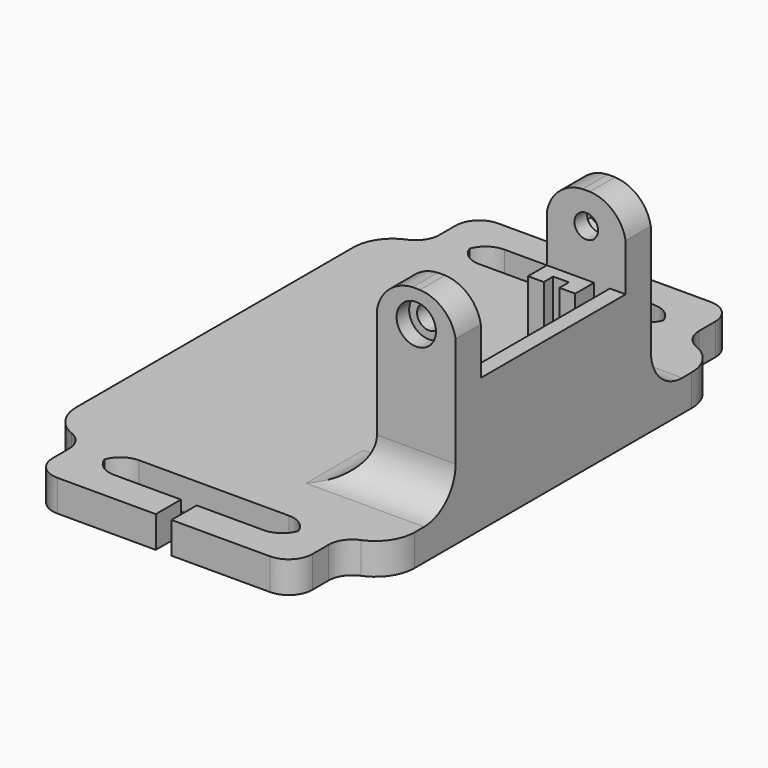
from build123d import *

# Parameters (mm, degrees)
F1_R          = 1.5
F2_DEPTH      = 4
F4_W          = 43
F4_H          = 54
F5_DEPTH      = 4
F6_R          = 5
F7_W          = 4
F7_H          = 4
F8_DEPTH      = 8
F8_DEPTH_BACK = 62
F9_W          = 4
F9_H          = 4
F10_DEPTH     = 25
F11_W         = 2
F11_H         = 4
F12_DEPTH     = 5
F11_H_2       = 15
F11_H_3       = 8
F11_H_4       = 1.5
F13_DEPTH     = 13
F14_DEPTH     = 7
F15_T1_DEPTH  = 3
F15_T3_DEPTH  = 3
F15_T5_DEPTH  = 2
F15_T7_DEPTH  = 4
F15_T12_DEPTH = 17
F15_T17_DEPTH = 17
F15_T22_DEPTH = 17
F15_T28_DEPTH = 9.5
F15_T33_DEPTH = 9.5
F15_T38_DEPTH = 17
F15_T45_DEPTH = 9.5
F15_T49_DEPTH = 10.5
F15_T56_DEPTH = 10.5
F15_T60_DEPTH = 9.5
F15_T63_DEPTH = 19
F16_R         = 2.5
F16_R_2       = 1.5
F17_DEPTH     = 2
F18_R         = 1.5
F19_DEPTH     = 2


# Not quite as in the source:
# - a fillet or chamfer that OpenCascade refuses, or shapes differently, is made with other operations: its cross-section is extruded or revolved along the edge and cut away or added


with BuildPart() as f2:
    # F1 (on offset) → F2 (new body)
    with BuildSketch(Plane.XZ.offset(11.5)):
        with BuildLine():
            Line((-10, 0), (0, 0))
            Line((0, 0), (0, 19))
            ThreePointArc((0, 19), (-1.5652731311, 21.7951628703), (-4.5336704997, 23))
            Line((-4.5336704997, 23), (-5, 23))
            Line((-5, 23), (-5.4663295003, 23))
            ThreePointArc((-5.4663295003, 23), (-8.4347268689, 21.7951628703), (-10, 19))
            Line((-10, 19), (-10, 0))
        make_face()
        with Locations((-5, 19)):
            Circle(F1_R, mode=Mode.SUBTRACT)
    extrude(amount=F2_DEPTH)


with BuildPart() as f3_1:
    # F3: instance of F2
    add(f2.part.mirror(Plane.XZ))


with BuildPart() as f2_1:
    add(f2.part)

    add(f3_1.part)  # F5 merges F3_1
    # F4 (on Top) → F5 (join)
    with BuildSketch(Plane.XY):
        with Locations((-21.5, 0)):
            Rectangle(F4_W, F4_H)
    extrude(amount=-F5_DEPTH)

    # F6
    f6_edges = [f2_1.edges().sort_by_distance(p)[0] for p in [
        (-5, -15.5, 0),
        (-5, 15.5, 0),
        (-10, 13.5, 0),
        (-10, -13.5, 0),
        (-43, 27, -2),
        (-43, -27, -2),
        (0, -27, -2),
        (0, 27, -2),
    ]]
    fillet(f6_edges, radius=F6_R)

    # F7 (on face) → F8 (join, two sides)
    with BuildSketch(Plane(origin=(0, 27, 0), x_dir=(-1, 0, 0), z_dir=(0, 1, 0))) as f8_sk:
        with Locations((36, -2)):
            Rectangle(F7_W, F7_H)
        with Locations((7, -2)):
            Rectangle(F7_W, F7_H)
    extrude(amount=F8_DEPTH)
    extrude(f8_sk.sketch, amount=-F8_DEPTH_BACK)

    # F9 (on face) → F10 (join)
    with BuildSketch(Plane.YZ.offset(-34)):
        with Locations((-33, -2)):
            Rectangle(F9_W, F9_H)
        with Locations((33, -2)):
            Rectangle(F9_W, F9_H)
    extrude(amount=F10_DEPTH)

    # F11 (on face) → F12 (cut)
    with BuildSketch(Plane.XY):
        with Locations((-21.5, -33)):
            Rectangle(F11_W, F11_H)
        with Locations((-21.5, 33)):
            Rectangle(F11_W, F11_H)
    extrude(amount=-F12_DEPTH, mode=Mode.SUBTRACT)

    # F11 (on face) → F13 (join)
    with BuildSketch(Plane.XY):
        with Locations((-1, 4)):
            Rectangle(F11_W, F11_H_2)
        with Locations((-1, -7.5)):
            Rectangle(F11_W, F11_H_3)
        Polygon((-6, -10), (-6, -11.5), (-4, -11.5), (-4, -8.5), (-6, -8.5), align=None)
        with Locations((-7, -10.75)):
            Rectangle(F11_W, F11_H_4)
        Polygon((-10, -8.5), (-10, -11.5), (-8, -11.5), (-8, -10), (-8, -8.5), align=None)
        Polygon((-8, 11.5), (-10, 11.5), (-10, 8.5), (-8, 8.5), (-8, 10), align=None)
        with Locations((-7, 10.75)):
            Rectangle(F11_W, F11_H_4)
        Polygon((-6, 8.5), (-4, 8.5), (-4, 11.5), (-6, 11.5), (-6, 10), align=None)
    extrude(amount=F13_DEPTH)

    # F11 (on face) → F14 (join)
    with BuildSketch(Plane.XY):
        Polygon((-4, -8.5), (-4, -11.5), (-2, -11.5), (-2, -3.5), (-2, 11.5), (-4, 11.5), (-4, 8.5), align=None)
    extrude(amount=F14_DEPTH)

    # F15: fillet of radius 3 on 22 edges, made by hand

    # F15_s2 → F15_t1 (join)
    with BuildSketch(Plane.XZ.offset(8.5)):
        with BuildLine():
            ThreePointArc((-13, 0), (-10.8786796564, 0.8786796564), (-10, 3))
            Line((-10, 3), (-10, 0))
            Line((-10, 0), (-13, 0))
        make_face()
    extrude(amount=F15_T1_DEPTH)

    # F15_s4 → F15_t3 (join)
    with BuildSketch(Plane.XZ.offset(-11.5)):
        with BuildLine():
            ThreePointArc((-13, 0), (-10.8786796564, 0.8786796564), (-10, 3))
            Line((-10, 3), (-10, 0))
            Line((-10, 0), (-13, 0))
        make_face()
    extrude(amount=F15_T3_DEPTH)

    # F15_s6 → F15_t5 (join)
    with BuildSketch(Plane.YZ.offset(-10)):
        with BuildLine():
            ThreePointArc((-5.5, 0), (-7.6213203436, 0.8786796564), (-8.5, 3))
            Line((-8.5, 3), (-8.5, 0))
            Line((-8.5, 0), (-5.5, 0))
        make_face()
        with BuildLine():
            ThreePointArc((5.5, 0), (7.6213203436, 0.8786796564), (8.5, 3))
            Line((8.5, 3), (8.5, 0))
            Line((8.5, 0), (5.5, 0))
        make_face()
    extrude(amount=F15_T5_DEPTH)

    # F15_s8 → F15_t7 (join)
    with BuildSketch(Plane.XY.offset(-4)):
        with BuildLine():
            ThreePointArc((-9, -30), (-9.8786796564, -27.8786796564), (-12, -27))
            Line((-12, -27), (-9, -27))
            Line((-9, -27), (-9, -30))
        make_face()
        with BuildLine():
            ThreePointArc((-31, -27), (-33.1213203436, -27.8786796564), (-34, -30))
            Line((-34, -30), (-34, -27))
            Line((-34, -27), (-31, -27))
        make_face()
        with BuildLine():
            ThreePointArc((-34, -28), (-33.1213203436, -30.1213203436), (-31, -31))
            Line((-31, -31), (-34, -31))
            Line((-34, -31), (-34, -28))
        make_face()
        with BuildLine():
            ThreePointArc((-12, -31), (-9.8786796564, -30.1213203436), (-9, -28))
            Line((-9, -28), (-9, -31))
            Line((-9, -31), (-12, -31))
        make_face()
        with BuildLine():
            ThreePointArc((-38, -29.4161984871), (-38.5125314072, -27.739147504), (-39.875, -26.6351240544))
            ThreePointArc((-39.875, -26.6351240544), (-38.9550863123, -26.9079333875), (-38, -27))
            Line((-38, -27), (-38, -29.4161984871))
        make_face()
        with BuildLine():
            ThreePointArc((-3.125, -26.6351240544), (-4.4874685928, -27.739147504), (-5, -29.4161984871))
            Line((-5, -29.4161984871), (-5, -27))
            ThreePointArc((-5, -27), (-4.0449136877, -26.9079333875), (-3.125, -26.6351240544))
        make_face()
        with BuildLine():
            ThreePointArc((-39.875, 26.6351240544), (-38.5125314072, 27.739147504), (-38, 29.4161984871))
            Line((-38, 29.4161984871), (-38, 27))
            ThreePointArc((-38, 27), (-38.9550863123, 26.9079333875), (-39.875, 26.6351240544))
        make_face()
        with BuildLine():
            ThreePointArc((-12, 27), (-9.8786796564, 27.8786796564), (-9, 30))
            Line((-9, 30), (-9, 27))
            Line((-9, 27), (-12, 27))
        make_face()
        with BuildLine():
            ThreePointArc((-5, 29.4161984871), (-4.4874685928, 27.739147504), (-3.125, 26.6351240544))
            ThreePointArc((-3.125, 26.6351240544), (-4.0449136877, 26.9079333875), (-5, 27))
            Line((-5, 27), (-5, 29.4161984871))
        make_face()
        with BuildLine():
            ThreePointArc((-34, 30), (-33.1213203436, 27.8786796564), (-31, 27))
            Line((-31, 27), (-34, 27))
            Line((-34, 27), (-34, 30))
        make_face()
        with BuildLine():
            ThreePointArc((-31, 31), (-33.1213203436, 30.1213203436), (-34, 28))
            Line((-34, 28), (-34, 31))
            Line((-34, 31), (-31, 31))
        make_face()
        with BuildLine():
            ThreePointArc((-9, 28), (-9.8786796564, 30.1213203436), (-12, 31))
            Line((-12, 31), (-9, 31))
            Line((-9, 31), (-9, 28))
        make_face()
    extrude(amount=F15_T7_DEPTH)


with BuildPart() as f15_tool10:
    # F15_s11 → F15_t12 (new body)
    with BuildSketch(Plane.YZ.offset(-0.5)):
        with BuildLine():
            ThreePointArc((-5.5, 0), (-7.6213203436, 0.8786796564), (-8.5, 3))
            Line((-8.5, 3), (-8.5, 0))
            Line((-8.5, 0), (-5.5, 0))
        make_face()
    extrude(amount=-F15_T12_DEPTH)

    split(bisect_by=Plane.YZ.offset(-6), keep=Keep.TOP)


with BuildPart() as f2_2:
    add(f2_1.part)

    # F15_t9: union F15_tool10
    add(f15_tool10.part)


with BuildPart() as f15_tool15:
    # F15_s16 → F15_t17 (new body)
    with BuildSketch(Plane.YZ.offset(-17.5)):
        with BuildLine():
            ThreePointArc((5.5, 0), (7.6213203436, 0.8786796564), (8.5, 3))
            Line((8.5, 3), (8.5, 0))
            Line((8.5, 0), (5.5, 0))
        make_face()
    extrude(amount=F15_T17_DEPTH)

    split(bisect_by=Plane.YZ.offset(-6), keep=Keep.TOP)


with BuildPart() as f2_3:
    add(f2_2.part)

    # F15_t14: union F15_tool15
    add(f15_tool15.part)


with BuildPart() as f15_tool20:
    # F15_s21 → F15_t22 (new body)
    with BuildSketch(Plane.YZ.offset(-13.5)):
        with BuildLine():
            ThreePointArc((5.5, 0), (7.6213203436, 0.8786796564), (8.5, 3))
            Line((8.5, 3), (8.5, 0))
            Line((8.5, 0), (5.5, 0))
        make_face()
    extrude(amount=F15_T22_DEPTH)

    split(bisect_by=Plane.YZ.offset(-10), keep=Keep.TOP)

    split(bisect_by=Plane.YZ.offset(-8), keep=Keep.BOTTOM)


with BuildPart() as f2_4:
    add(f2_3.part)

    # F15_t19: union F15_tool20
    add(f15_tool20.part)


with BuildPart() as f15_tool26:
    # F15_s27 → F15_t28 (new body)
    with BuildSketch(Plane.YZ.offset(-6)):
        with BuildLine():
            ThreePointArc((5.5, 0), (7.6213203436, 0.8786796564), (8.5, 3))
            Line((8.5, 3), (8.5, 0))
            Line((8.5, 0), (5.5, 0))
        make_face()
    extrude(amount=F15_T28_DEPTH)

    split(bisect_by=Plane.YZ, keep=Keep.BOTTOM)


with BuildPart() as f2_5:
    add(f2_4.part)

    # F15_t25: union F15_tool26
    add(f15_tool26.part)


with BuildPart() as f15_tool31:
    # F15_s32 → F15_t33 (new body)
    with BuildSketch(Plane.YZ.offset(3.5)):
        with BuildLine():
            ThreePointArc((-5.5, 0), (-7.6213203436, 0.8786796564), (-8.5, 3))
            Line((-8.5, 3), (-8.5, 0))
            Line((-8.5, 0), (-5.5, 0))
        make_face()
    extrude(amount=-F15_T33_DEPTH)

    split(bisect_by=Plane.YZ, keep=Keep.BOTTOM)


with BuildPart() as f2_6:
    add(f2_5.part)

    # F15_t30: union F15_tool31
    add(f15_tool31.part)


with BuildPart() as f15_tool36:
    # F15_s37 → F15_t38 (new body)
    with BuildSketch(Plane.YZ.offset(3.5)):
        with BuildLine():
            ThreePointArc((-5.5, 0), (-7.6213203436, 0.8786796564), (-8.5, 3))
            Line((-8.5, 3), (-8.5, 0))
            Line((-8.5, 0), (-5.5, 0))
        make_face()
    extrude(amount=-F15_T38_DEPTH)

    split(bisect_by=Plane.YZ.offset(-8), keep=Keep.BOTTOM)

    split(bisect_by=Plane.YZ.offset(-10), keep=Keep.TOP)


with BuildPart() as f2_7:
    add(f2_6.part)

    # F15_t35: union F15_tool36
    add(f15_tool36.part)


with BuildPart() as f15_tool43:
    # F15_s44 → F15_t45 (new body)
    with BuildSketch(Plane.YZ.offset(-8)):
        with BuildLine():
            ThreePointArc((-5.5, 0), (-7.6213203436, 0.8786796564), (-8.5, 3))
            Line((-8.5, 3), (-8.5, 0))
            Line((-8.5, 0), (-5.5, 0))
        make_face()
    extrude(amount=-F15_T45_DEPTH)

    split(bisect_by=Plane.YZ.offset(-10), keep=Keep.BOTTOM)


with BuildPart() as f15_tool47:
    # F15_s48 → F15_t49 (new body)
    with BuildSketch(Plane.XZ.offset(1)):
        with BuildLine():
            ThreePointArc((-13, 0), (-10.8786796564, 0.8786796564), (-10, 3))
            Line((-10, 3), (-10, 0))
            Line((-10, 0), (-13, 0))
        make_face()
    extrude(amount=F15_T49_DEPTH)

    split(bisect_by=Plane.XZ.offset(8.5), keep=Keep.BOTTOM)


with BuildPart() as f15_tool43_1:
    add(f15_tool43.part)

    # F15_t51: intersect F15_tool47
    add(f15_tool47.part, mode=Mode.INTERSECT)


with BuildPart() as f2_8:
    add(f2_7.part)

    # F15_t41: union F15_tool43
    add(f15_tool43_1.part)


with BuildPart() as f15_tool54:
    # F15_s55 → F15_t56 (new body)
    with BuildSketch(Plane.XZ.offset(-11.5)):
        with BuildLine():
            ThreePointArc((-13, 0), (-10.8786796564, 0.8786796564), (-10, 3))
            Line((-10, 3), (-10, 0))
            Line((-10, 0), (-13, 0))
        make_face()
    extrude(amount=F15_T56_DEPTH)

    split(bisect_by=Plane.XZ.offset(-8.5), keep=Keep.TOP)


with BuildPart() as f15_tool58:
    # F15_s59 → F15_t60 (new body)
    with BuildSketch(Plane.YZ.offset(-17.5)):
        with BuildLine():
            ThreePointArc((5.5, 0), (7.6213203436, 0.8786796564), (8.5, 3))
            Line((8.5, 3), (8.5, 0))
            Line((8.5, 0), (5.5, 0))
        make_face()
    extrude(amount=F15_T60_DEPTH)

    split(bisect_by=Plane.YZ.offset(-10), keep=Keep.BOTTOM)


with BuildPart() as f15_tool54_1:
    add(f15_tool54.part)

    # F15_t62: intersect F15_tool58
    add(f15_tool58.part, mode=Mode.INTERSECT)


with BuildPart() as f2_9:
    add(f2_8.part)

    # F15_t52: union F15_tool54
    add(f15_tool54_1.part)

    # F15_s64 → F15_t63 (cut)
    with BuildSketch(Plane.XY.offset(-11.5)):
        with BuildLine():
            ThreePointArc((-5, -32), (-5.8786796564, -34.1213203436), (-8, -35))
            Line((-8, -35), (-5, -35))
            Line((-5, -35), (-5, -32))
        make_face()
        with BuildLine():
            ThreePointArc((-35, -35), (-37.1213203436, -34.1213203436), (-38, -32))
            Line((-38, -32), (-38, -35))
            Line((-38, -35), (-35, -35))
        make_face()
        with BuildLine():
            ThreePointArc((-38, 32), (-37.1213203436, 34.1213203436), (-35, 35))
            Line((-35, 35), (-38, 35))
            Line((-38, 35), (-38, 32))
        make_face()
        with BuildLine():
            ThreePointArc((-8, 35), (-5.8786796564, 34.1213203436), (-5, 32))
            Line((-5, 32), (-5, 35))
            Line((-5, 35), (-8, 35))
        make_face()
    extrude(amount=F15_T63_DEPTH, mode=Mode.SUBTRACT)

    # F16 (on face) → F17 (cut)
    with BuildSketch(Plane.XZ.offset(15.5)):
        with Locations((-5, 19)):
            Circle(F16_R)
        with Locations((-5, 19)):
            Circle(F16_R_2, mode=Mode.SUBTRACT)
    extrude(amount=-F17_DEPTH, mode=Mode.SUBTRACT)

    # F18 (on face) → F19 (cut)
    with BuildSketch(Plane(origin=(0, 15.5, 0), x_dir=(-1, 0, 0), z_dir=(0, 1, 0))):
        Polygon((7.6, 17.4988893001), (7.6, 20.5011106999), (5, 22.0022213998), (2.4, 20.5011106999), (2.4, 17.4988893001), (5, 15.9977786002), align=None)
        with Locations((5, 19)):
            Circle(F18_R, mode=Mode.SUBTRACT)
    extrude(amount=-F19_DEPTH, mode=Mode.SUBTRACT)


solid = f2_9.part
